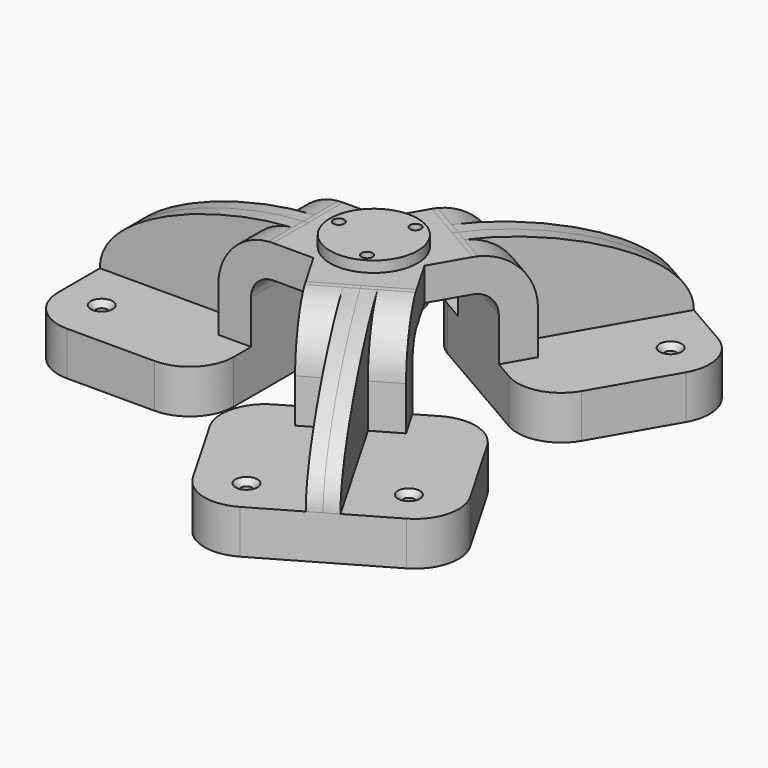
from build123d import *

# Parameters (mm, degrees)
F1_DEPTH        = 63.5
F0_W            = 25.4
F0_H            = 19.0499989867
F2_DEPTH        = 25.4
F3_DEPTH        = 7.9375
F6_D            = 6.35
F6_CSINK_D      = 12.7
F6_CSINK_ANGLE  = 90
F7_COUNT        = 3
F9_D            = 6.35
F9_COPIES_COUNT = 3
F10_R           = 25.4


# Not quite as in the source:
# - a pattern or mirror of a feature is missing from the dataset's text; its kind, count and spacing are read off the source's solid


with BuildPart() as f1:
    # F0 (on Front) → F1 (new body, symmetric)
    with BuildSketch(Plane.XZ):
        Polygon((50.8, -12.7), (50.8, 12.7), (31.7500010133, 12.7), (-50.8, 12.7), (-50.8, -12.7), align=None)
    extrude(amount=F1_DEPTH, both=True)

    # F0 (on Front) → F2 (join, symmetric)
    with BuildSketch(Plane.XZ):
        with BuildLine():
            Line((31.7500010133, 12.7), (50.8, 12.7))
            Line((50.8, 12.7), (50.8, 38.1))
            ThreePointArc((50.8, 38.1), (54.5197438789, 47.0802561211), (63.5, 50.8))
            Line((63.5, 50.8), (76.2, 50.8))
            Line((76.2, 50.8), (76.2, 69.8499989867))
            Line((76.2, 69.8499989867), (63.5, 69.8499989867))
            add(Edge.make_bspline(
                [(60.7424728123, 69.7300249678), (61.6706362679, 69.7791364012), (62.5900608791, 69.8191720775), (63.5, 69.8499989867)],
                knots=[125.2378350903, 125.2378350903, 125.2378350903, 125.2378350903, 127.791284461, 127.791284461, 127.791284461, 127.791284461], degree=3))
            ThreePointArc((60.7424728123, 69.7300249678), (40.0947236603, 59.5535655573), (31.7500010133, 38.1))
            Line((31.7500010133, 38.1), (31.7500010133, 12.7))
        make_face()
        with Locations((88.9, 60.3249994934)):
            Rectangle(F0_W, F0_H)
    extrude(amount=F2_DEPTH, both=True)

    # F0 (on Front) → F3 (join, symmetric)
    with BuildSketch(Plane.XZ):
        with BuildLine():
            Line((-50.8, 12.7), (31.7500010133, 12.7))
            Line((31.7500010133, 12.7), (31.7500010133, 38.1))
            ThreePointArc((31.7500010133, 38.1), (40.0947236603, 59.5535655573), (60.7424728123, 69.7300249678))
            add(Edge.make_bspline(
                [(-50.8, 12.7), (-51.3257578554, 43.0802353164), (15.219274615, 67.3212795022), (60.7424728123, 69.7300249678)],
                knots=[0, 0, 0, 0, 125.2378350903, 125.2378350903, 125.2378350903, 125.2378350903], degree=3))
        make_face()
    extrude(amount=F3_DEPTH, both=True)

    # F0 (on Front) → F4 (revolve)
    with BuildSketch(Plane.XZ):
        Polygon((101.6, 69.8499989867), (101.6, 50.8), (101.6, 44.45), (127, 44.45), (127, 76.2), (101.6, 76.2), align=None)
    revolve(axis=Axis((101.6, 0, 60.325), (0, 0, -1)))

    # F6 (through all)
    with Locations(Plane.XY.offset(12.7)):
        with Locations((-27.541898191, -35.71875), (-27.541898191, 38.6316925287)):
            CounterSinkHole(F6_D / 2, F6_CSINK_D / 2, counter_sink_angle=F6_CSINK_ANGLE)

    # F7: F1 ×3 about axis
    f7_axis = Axis((101.6, 0, 60.325), (0, 0, -1))


with BuildPart() as f1_1:
    add(f1.part)
    for i in range(1, F7_COUNT):
        add(f1.part.rotate(f7_axis, i * 360 / F7_COUNT))

    # F9 (through all)
    with Locations(Plane.XY.offset(76.2)):
        with Locations((81.3262090087, 0)):
            f9 = Hole(F9_D / 2)

    # F9_copies: F9 ×3 about axis
    f9_copies_axis = Axis((101.6, 0, 0), (0, 0, 1))
    for i in range(1, F9_COPIES_COUNT):
        add(f9.rotate(f9_copies_axis, i * 360 / F9_COPIES_COUNT), mode=Mode.SUBTRACT)

    # F10
    f10_edges = [f1_1.edges().sort_by_distance(p)[0] for p in [
        (-50.8, -63.5, 0),
        (122.807387, -163.732272, 0),
        (232.792613, -100.232272, 0),
        (232.792613, 100.232272, 0),
        (181.992613, 12.244091, 0),
        (181.992613, -12.244091, 0),
        (50.8, -63.5, 0),
        (122.807387, 163.732272, 0),
        (72.007387, 75.744091, 0),
        (72.007387, -75.744091, 0),
        (50.8, 63.5, 0),
        (-50.8, 63.5, 0),
    ]]
    fillet(f10_edges, radius=F10_R)


solid = f1_1.part
